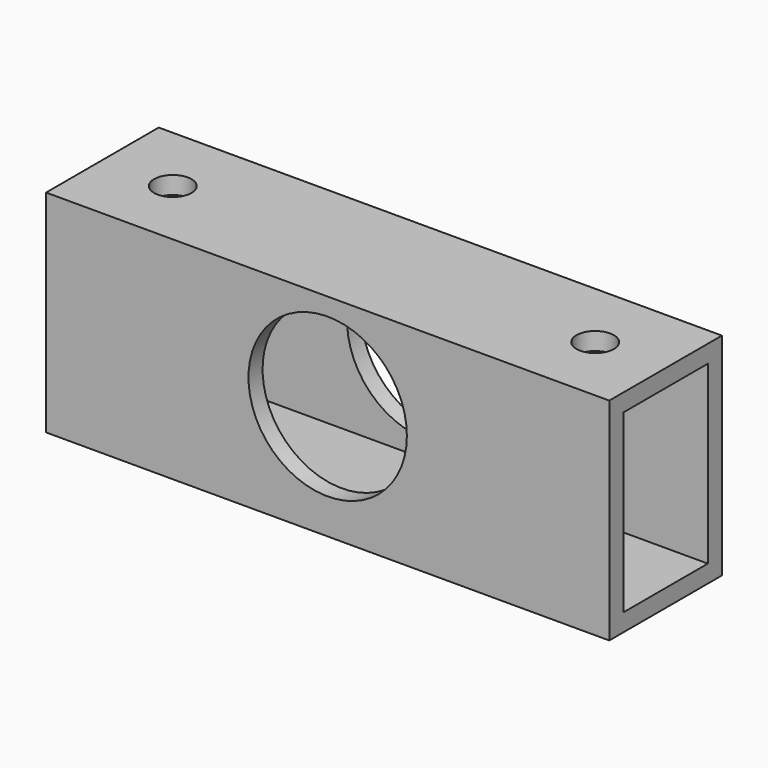
from build123d import *

# Parameters (mm, degrees)
F0_W          = 101.6
F0_H          = 25.4
F0_R          = 3.3782
F1_DEPTH      = 38.1
F2_R          = 14.2875
F3_DEPTH      = 25.4
F4_W          = 19.05
F4_H          = 31.75
F5_DEPTH      = 50.801
F5_DEPTH_BACK = 50.801


# Not quite as in the source:
# - a feature names something its author has since deleted; it is built from what else it names


with BuildPart() as f1:
    # F0 (on Top) → F1 (new body)
    with BuildSketch(Plane.XY):
        Rectangle(F0_W, F0_H)
        with Locations((-38.1, 0)):
            Circle(F0_R, mode=Mode.SUBTRACT)
        with Locations((38.1, 0)):
            Circle(F0_R, mode=Mode.SUBTRACT)
    extrude(amount=F1_DEPTH)

    # F2 (on face) → F3 (cut)
    with BuildSketch(Plane.XZ.offset(12.7)):
        with Locations((0, 20.6375)):
            Circle(F2_R)
    extrude(amount=-F3_DEPTH, mode=Mode.SUBTRACT)

    # F4 (on Right) → F5 (cut, two sides)
    with BuildSketch(Plane.YZ) as f5_sk:
        with Locations((0, 19.05)):
            Rectangle(F4_W, F4_H)
    extrude(amount=-F5_DEPTH, mode=Mode.SUBTRACT)
    extrude(f5_sk.sketch, amount=F5_DEPTH_BACK, mode=Mode.SUBTRACT)


solid = f1.part
